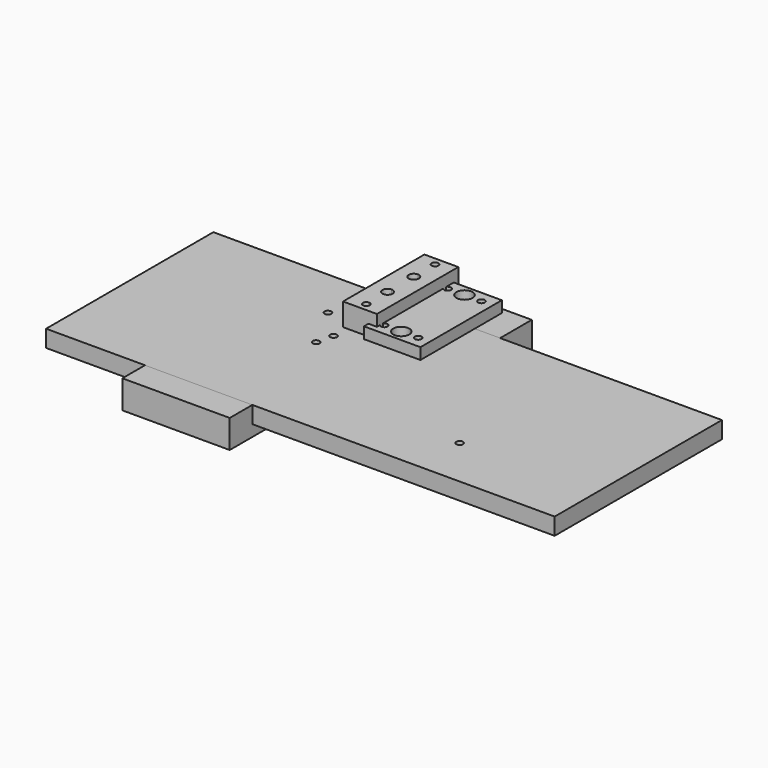
from build123d import *

# Parameters (mm, degrees)
F0_W             = 450
F0_H             = 155
F1_DEPTH         = 15
F4_W             = 95
F4_H             = 45
F5_DEPTH         = 25
F7_DEPTH         = 20
F9_D             = 6
F9_DEPTH         = 25
F9_TIP           = 1.8025818571
F11_D            = 8.8
F11_DEPTH        = 25
F11_CBORE_D      = 14.25
F11_CBORE_DEPTH  = 8
F11_TIP          = 2.6437867237
F13_R            = 3
F14_DEPTH        = 15
F15_W            = 50
F15_H            = 90
F16_DEPTH        = 10
F18_D            = 8.8
F18_DEPTH        = 15.75
F18_CBORE_D      = 14.25
F18_CBORE_DEPTH  = 8
F18_TIP          = 2.6437867237
F19_D            = 8.8
F19_DEPTH        = 50
F19_TIP          = 2.6437867237
F21_D            = 8.8
F21_DEPTH        = 50
F21_TIP          = 2.6437867237
F22_D            = 15
F22_DEPTH        = 50
F22_TIP          = 4.5064546427
F23_W            = 450
F23_H            = 185
F24_DEPTH        = 15
F25_D            = 6
F25_DEPTH        = 50
F25_TIP          = 1.8025818571
F27_D            = 6
F27_DEPTH        = 50
F27_TIP          = 1.8025818571
F27_2_D          = 6
F27_2_DEPTH      = 50
F27_2_TIP        = 1.8025818571
F28_D            = 15
F28_DEPTH        = 50
F28_TIP          = 4.5064546427
F29_D            = 6
F29_DEPTH        = 50
F29_TIP          = 1.8025818571
F29_ON_F15_D     = 6
F29_ON_F15_DEPTH = 50
F29_ON_F15_TIP   = 1.8025818571
F30_D            = 9
F30_DEPTH        = 50
F30_TIP          = 2.7038727856


# Not quite as in the source:
# - a feature of the source that left no trace in its solid (it failed there, or was rolled back) is left out


with BuildPart() as f1:
    # F0 (on Top) → F1 (new body)
    with BuildSketch(Plane.XY):
        with Locations((-105, 52.5)):
            Rectangle(F0_W, F0_H)
    extrude(amount=-F1_DEPTH)

    # F9
    with Locations(Plane.XY):
        with Locations((-192.93, 95.41), (-168.18, 70.66), (-171.71, 55.81)):
            Hole(F9_D / 2, depth=F9_DEPTH)
            with Locations((0, 0, -(F9_DEPTH + F9_TIP / 2))):  # 118° drill point
                Cone(0, F9_D / 2, F9_TIP, mode=Mode.SUBTRACT)

    # F11
    with Locations(Plane(origin=(0, 0, -15), x_dir=(1, 0, 0), z_dir=(0, 0, -1))):
        with Locations((-180.9, -65), (-198.58, -82.68)):
            CounterBoreHole(F11_D / 2, F11_CBORE_D / 2, F11_CBORE_DEPTH, depth=F11_DEPTH)
            with Locations((0, 0, -(F11_DEPTH + F11_TIP / 2))):  # 118° drill point
                Cone(0, F11_D / 2, F11_TIP, mode=Mode.SUBTRACT)

    # F19
    with Locations(Plane.XY):
        with Locations((-123.7564434702, 90)):
            Hole(F19_D / 2, depth=F19_DEPTH)
            with Locations((0, 0, -(F19_DEPTH + F19_TIP / 2))):  # 118° drill point
                Cone(0, F19_D / 2, F19_TIP, mode=Mode.SUBTRACT)

    # F21
    with Locations(Plane.XY):
        with Locations((-73.7564434702, 57)):
            Hole(F21_D / 2, depth=F21_DEPTH)
            with Locations((0, 0, -(F21_DEPTH + F21_TIP / 2))):  # 118° drill point
                Cone(0, F21_D / 2, F21_TIP, mode=Mode.SUBTRACT)

    # F22
    with Locations(Plane.XY):
        with Locations((-195, -13)):
            Hole(F22_D / 2, depth=F22_DEPTH)
            with Locations((0, 0, -(F22_DEPTH + F22_TIP / 2))):  # 118° drill point
                Cone(0, F22_D / 2, F22_TIP, mode=Mode.SUBTRACT)

    # F27
    with Locations(Plane.XY):
        with Locations((0, 0)):
            Hole(F27_D / 2, depth=F27_DEPTH)
            with Locations((0, 0, -(F27_DEPTH + F27_TIP / 2))):  # 118° drill point
                Cone(0, F27_D / 2, F27_TIP, mode=Mode.SUBTRACT)

    # F29 on F15
    with Locations(Plane.XY):
        with Locations((-138.7564434702, 90), (-108.7564434702, 90)):
            Hole(F29_ON_F15_D / 2, depth=F29_ON_F15_DEPTH)
            with Locations((0, 0, -(F29_ON_F15_DEPTH + F29_ON_F15_TIP / 2))):  # 118° drill point
                Cone(0, F29_ON_F15_D / 2, F29_ON_F15_TIP, mode=Mode.SUBTRACT)


with BuildPart() as f5:
    # F4 (on face) → F5 (new body)
    with BuildSketch(Plane.XY):
        with Locations((-195, -47.5)):
            Rectangle(F4_W, F4_H)
    extrude(amount=-F5_DEPTH)


with BuildPart() as f5b:
    # F4 (on face) → F5, piece 2 (new body)
    with BuildSketch(Plane.XY):
        with Locations((-123.7564434702, 152.5)):
            Rectangle(F4_W, F4_H)
    extrude(amount=-F5_DEPTH)

    # F28
    with Locations(Plane.XY):
        with Locations((-123.7564434702, 143.6025403784)):
            Hole(F28_D / 2, depth=F28_DEPTH)
            with Locations((0, 0, -(F28_DEPTH + F28_TIP / 2))):  # 118° drill point
                Cone(0, F28_D / 2, F28_TIP, mode=Mode.SUBTRACT)

    # F29
    with Locations(Plane.XY):
        with Locations((-108.7564434702, 160), (-138.7564434702, 160)):
            Hole(F29_D / 2, depth=F29_DEPTH)
            with Locations((0, 0, -(F29_DEPTH + F29_TIP / 2))):  # 118° drill point
                Cone(0, F29_D / 2, F29_TIP, mode=Mode.SUBTRACT)

    # F30
    with Locations(Plane.XY):
        with Locations((-123.7564434702, 160)):
            Hole(F30_D / 2, depth=F30_DEPTH)
            with Locations((0, 0, -(F30_DEPTH + F30_TIP / 2))):  # 118° drill point
                Cone(0, F30_D / 2, F30_TIP, mode=Mode.SUBTRACT)


with BuildPart() as f7:
    # F6 (on face) → F7 (new body)
    with BuildSketch(Plane.XY):
        Polygon((-141.2564434702, 175), (-171.2564434702, 175), (-171.2564434702, 85), (-141.2564434702, 85), (-141.2564434702, 168), align=None)
        with BuildLine():
            ThreePointArc((-153.2564434702, 92), (-158.3777638137, 89.8786796564), (-156.2564434702, 95))
            ThreePointArc((-156.2564434702, 95), (-154.1351231266, 94.1213203436), (-153.2564434702, 92))
        make_face(mode=Mode.SUBTRACT)
        with BuildLine():
            ThreePointArc((-156.2564434702, 111), (-160.7564434702, 115.5), (-156.2564434702, 120))
            ThreePointArc((-156.2564434702, 120), (-153.0744629548, 118.6819805153), (-151.7564434702, 115.5))
            ThreePointArc((-151.7564434702, 115.5), (-153.0744629548, 112.3180194847), (-156.2564434702, 111))
        make_face(mode=Mode.SUBTRACT)
        with BuildLine():
            ThreePointArc((-156.2564434702, 140), (-160.7564434702, 144.5), (-156.2564434702, 149))
            ThreePointArc((-156.2564434702, 149), (-153.0744629548, 147.6819805153), (-151.7564434702, 144.5))
            ThreePointArc((-151.7564434702, 144.5), (-153.0744629548, 141.3180194847), (-156.2564434702, 140))
        make_face(mode=Mode.SUBTRACT)
        with BuildLine():
            ThreePointArc((-156.2564434702, 165), (-158.3777638137, 170.1213203436), (-153.2564434702, 168))
            ThreePointArc((-153.2564434702, 168), (-154.1351231266, 165.8786796564), (-156.2564434702, 165))
        make_face(mode=Mode.SUBTRACT)
    extrude(amount=F7_DEPTH)


with BuildPart() as f14:
    # F13 (on face) → F14 (new body)
    with BuildSketch(Plane.XY):
        Polygon((-148.7564434702, 170), (-148.7564434702, 130), (-98.7564434702, 130), (-98.7564434702, 170), (-123.7564434702, 170), align=None)
        with BuildLine():
            ThreePointArc((-116.2564434702, 143.6025403784), (-129.0597443291, 138.2992395195), (-123.7564434702, 151.1025403784))
            ThreePointArc((-123.7564434702, 151.1025403784), (-118.4531426113, 148.9058412373), (-116.2564434702, 143.6025403784))
        make_face(mode=Mode.SUBTRACT)
        with Locations((-138.7564434702, 160)):
            Circle(F13_R, mode=Mode.SUBTRACT)
        with BuildLine():
            ThreePointArc((-128.2564434702, 160), (-126.9384239855, 163.1819805153), (-123.7564434702, 164.5))
            ThreePointArc((-123.7564434702, 164.5), (-120.5744629548, 163.1819805153), (-119.2564434702, 160))
            ThreePointArc((-119.2564434702, 160), (-120.5744629548, 156.8180194847), (-123.7564434702, 155.5))
            ThreePointArc((-123.7564434702, 155.5), (-126.9384239855, 156.8180194847), (-128.2564434702, 160))
        make_face(mode=Mode.SUBTRACT)
        with BuildLine():
            ThreePointArc((-105.7564434702, 160), (-108.7564434702, 157), (-111.7564434702, 160))
            ThreePointArc((-111.7564434702, 160), (-108.7564434702, 163), (-105.7564434702, 160))
        make_face(mode=Mode.SUBTRACT)
    extrude(amount=-F14_DEPTH)


with BuildPart() as f16:
    # F15 (on face) → F16 (new body)
    with BuildSketch(Plane.XY):
        with Locations((-123.7564434702, 125)):
            Rectangle(F15_W, F15_H)
        with BuildLine():
            ThreePointArc((-138.7564434702, 93), (-136.6351231266, 92.1213203436), (-135.7564434702, 90))
            ThreePointArc((-135.7564434702, 90), (-140.8777638137, 87.8786796564), (-138.7564434702, 93))
        make_face(mode=Mode.SUBTRACT)
        with BuildLine():
            ThreePointArc((-119.2564434702, 90), (-123.7564434702, 85.5), (-128.2564434702, 90))
            ThreePointArc((-128.2564434702, 90), (-126.9384239855, 93.1819805153), (-123.7564434702, 94.5))
            ThreePointArc((-123.7564434702, 94.5), (-120.5744629548, 93.1819805153), (-119.2564434702, 90))
        make_face(mode=Mode.SUBTRACT)
        with BuildLine():
            ThreePointArc((-105.7564434702, 90), (-108.7564434702, 87), (-111.7564434702, 90))
            ThreePointArc((-111.7564434702, 90), (-110.8777638137, 92.1213203436), (-108.7564434702, 93))
            ThreePointArc((-108.7564434702, 93), (-106.6351231266, 92.1213203436), (-105.7564434702, 90))
        make_face(mode=Mode.SUBTRACT)
        with BuildLine():
            ThreePointArc((-135.7564434702, 160), (-136.6351231266, 157.8786796564), (-138.7564434702, 157))
            ThreePointArc((-138.7564434702, 157), (-140.8777638137, 162.1213203436), (-135.7564434702, 160))
        make_face(mode=Mode.SUBTRACT)
        with BuildLine():
            ThreePointArc((-119.2564434702, 160), (-120.5744629548, 156.8180194847), (-123.7564434702, 155.5))
            ThreePointArc((-123.7564434702, 155.5), (-126.9384239855, 163.1819805153), (-119.2564434702, 160))
        make_face(mode=Mode.SUBTRACT)
        with BuildLine():
            ThreePointArc((-105.7564434702, 160), (-106.6351231266, 157.8786796564), (-108.7564434702, 157))
            ThreePointArc((-108.7564434702, 157), (-110.8777638137, 162.1213203436), (-105.7564434702, 160))
        make_face(mode=Mode.SUBTRACT)
    extrude(amount=F16_DEPTH)

    # F18
    with Locations(Plane.XY.offset(10)):
        with Locations((-123.7564434702, 160), (-123.7564434702, 90)):
            CounterBoreHole(F18_D / 2, F18_CBORE_D / 2, F18_CBORE_DEPTH, depth=F18_DEPTH)
            with Locations((0, 0, -(F18_DEPTH + F18_TIP / 2))):  # 118° drill point
                Cone(0, F18_D / 2, F18_TIP, mode=Mode.SUBTRACT)


with BuildPart() as f24:
    # F23 (on face) → F24 (new body)
    with BuildSketch(Plane.XY):
        with Locations((-105, 47.5)):
            Rectangle(F23_W, F23_H)
    extrude(amount=-F24_DEPTH)

    # F25
    with Locations(Plane.XY):
        with Locations((-192.93, 95.41), (-168.18, 70.66), (-171.71, 55.81)):
            Hole(F25_D / 2, depth=F25_DEPTH)
            with Locations((0, 0, -(F25_DEPTH + F25_TIP / 2))):  # 118° drill point
                Cone(0, F25_D / 2, F25_TIP, mode=Mode.SUBTRACT)

    # F27#2
    with Locations(Plane.XY):
        with Locations((0, 0)):
            Hole(F27_2_D / 2, depth=F27_2_DEPTH)
            with Locations((0, 0, -(F27_2_DEPTH + F27_2_TIP / 2))):  # 118° drill point
                Cone(0, F27_2_D / 2, F27_2_TIP, mode=Mode.SUBTRACT)


solid = Compound([f1.part, f5.part, f5b.part, f7.part, f14.part, f16.part, f24.part])
